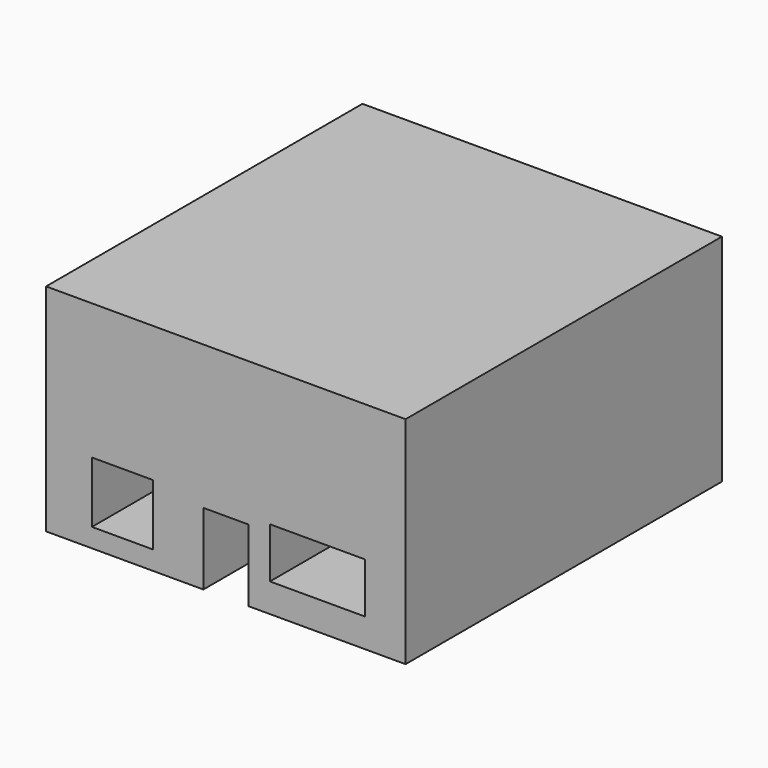
from build123d import *

# Parameters (mm, degrees)
F0_W     = 172.72
F0_H     = 172.72
F0_W_2   = 269.24
F0_H_2   = 142.24
F2_DEPTH = 1117.6
F0_W_3   = 228.6
F0_H_3   = 101.6
F3_DEPTH = 38.1
F0_W_4   = 127
F0_H_4   = 127


# Not quite as in the source:
# - the program builds the solid bodies; features that only make, move or delete a surface that nothing else refers to are left out


with BuildPart() as f2:
    # F0 (on Front) → F2 (new body)
    with BuildSketch(Plane.XZ):
        Polygon((508, 0), (0, 0), (-508, 0), (-508, -609.6), (-67.5734877586, -609.6), (-63.5, -609.6), (-63.5, -406.4), (63.5, -406.4), (63.5, -609.6), (508, -609.6), align=None)
        with Locations((-292.1, -469.9)):
            Rectangle(F0_W, F0_H, mode=Mode.SUBTRACT)
        with Locations((259.2723690559, -457.2)):
            Rectangle(F0_W_2, F0_H_2, mode=Mode.SUBTRACT)
    extrude(amount=F2_DEPTH)

    # F0 (on Front) → F3 (join)
    with BuildSketch(Plane.XZ):
        with Locations((259.2723690559, -457.2)):
            Rectangle(F0_W_2, F0_H_2)
        with Locations((259.2723690559, -457.2)):
            Rectangle(F0_W_3, F0_H_3, mode=Mode.SUBTRACT)
    extrude(amount=F3_DEPTH)


with BuildPart() as f3:
    # F0 (on Front) → F3, piece 2 (new body)
    with BuildSketch(Plane.XZ):
        with Locations((-292.1, -469.9)):
            Rectangle(F0_W_4, F0_H_4)
    extrude(amount=F3_DEPTH)


solid = Compound([f2.part, f3.part])
